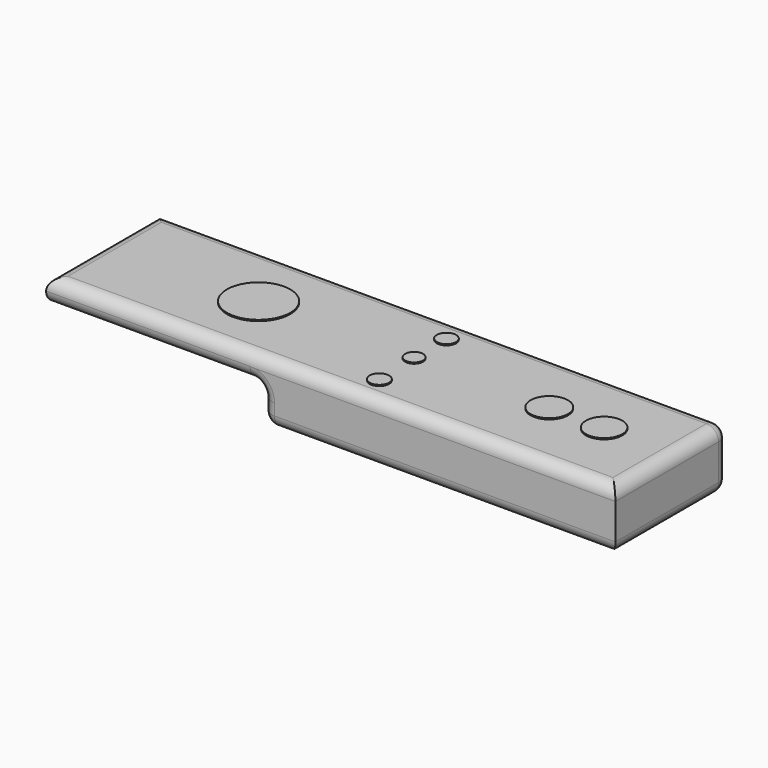
from build123d import *

# Parameters (mm, degrees)
F0_W          = 237.3272180557
F0_H          = 58.8164292276
F1_DEPTH      = 10
F2_W          = 147.2023129463
F2_H          = 58.8164292276
F3_DEPTH      = 15
F4_F1_R       = 5.08
F4_F2_R       = 5.08
F5_W          = 55.2143082023
F5_H          = 22.0865048468
F6_DEPTH      = 4
F7_T1_DEPTH   = 46.9058521388
F7_T3_DEPTH   = 80.0336554942
F9_R          = 13.2118644906
F10_DEPTH     = 0.5
F12_R         = 4.0488978151
F13_DEPTH     = 0.5
F12_R_2       = 3.7300649458
F12_R_3       = 4.0152102199
F12_R_4       = 7.8029945449
F12_R_5       = 7.5839402098
F14_T1_DEPTH  = 262.7272180557
F15_T1_DEPTH  = 66.4364292276
F15_T3_DEPTH  = 262.7272180557
F15_T5_DEPTH  = 14.84
F15_S9_W      = 5.08
F15_S9_H      = 5.08
F15_T10_DEPTH = 5.08
F15_T14_ANGLE = 89.9999999979
F16_T1_DEPTH  = 74.0564292276


# Not quite as in the source:
# - a fillet or chamfer that OpenCascade refuses, or shapes differently, is made with other operations: its cross-section is extruded or revolved along the edge and cut away or added


with BuildPart() as f1:
    # F0 (on Top) → F1 (new body)
    with BuildSketch(Plane.XY):
        Rectangle(F0_W, F0_H)
    extrude(amount=F1_DEPTH)

    # F2 (on face) → F3 (join)
    with BuildSketch(Plane(origin=(0, 0, 0), x_dir=(1, 0, 0), z_dir=(0, 0, -1))):
        with Locations((45.0624525547, 0)):
            Rectangle(F2_W, F2_H)
    extrude(amount=F3_DEPTH)

    # F4: fillet of radius 5.08 on 7 edges, made by hand

    # F4_f1
    f4_f1_edges = [f1.edges().sort_by_distance(p)[0] for p in [
        (-28.5387039185, 0, 0),
    ]]
    fillet(f4_f1_edges, radius=F4_F1_R)

    # F4_f2
    f4_f2_edges = [f1.edges().sort_by_distance(p)[0] for p in [
        (-28.5387039185, -29.4082146138, -10.04),
        (-28.5387039185, 29.4082146138, -10.04),
        (-28.5387039185, 0, -15),
        (45.0624525547, 29.4082146138, -15),
        (118.6636090279, 0, -15),
        (45.0624525547, -29.4082146138, -15),
        (-30.02660147, 29.4082146138, -1.4878975516),
        (-30.02660147, -29.4082146138, -1.4878975516),
    ]]
    fillet(f4_f2_edges, radius=F4_F2_R)

    # F5 (on face) → F6 (join)
    with BuildSketch(Plane(origin=(0, 0, 0), x_dir=(1, 0, 0), z_dir=(0, 0, -1))):
        with Locations((-83.400927484, 0)):
            Rectangle(F5_W, F5_H)
    extrude(amount=F6_DEPTH)

    # F7: fillet of radius 5.08 on 4 edges, made by hand

    # F7_s2 → F7_t1 (cut)
    with BuildSketch(Plane.XZ.offset(-23.4529260694)):
        with BuildLine():
            ThreePointArc((-55.7937733829, 0), (-57.5701673512, -2.8755530587), (-60.7576428413, -4))
            Line((-60.7576428413, -4), (-55.7937733829, -4))
            Line((-55.7937733829, -4), (-55.7937733829, 0))
        make_face()
        with BuildLine():
            ThreePointArc((-111.0080815852, 0), (-109.2316876169, -2.8755530587), (-106.0442121268, -4))
            Line((-106.0442121268, -4), (-111.0080815852, -4))
            Line((-111.0080815852, -4), (-111.0080815852, 0))
        make_face()
    extrude(amount=F7_T1_DEPTH, mode=Mode.SUBTRACT)

    # F7_s4 → F7_t3 (cut)
    with BuildSketch(Plane.YZ.offset(-123.4177552312)):
        with BuildLine():
            ThreePointArc((-11.0432524234, 0), (-9.2668584551, -2.8755530587), (-6.079382965, -4))
            Line((-6.079382965, -4), (-11.0432524234, -4))
            Line((-11.0432524234, -4), (-11.0432524234, 0))
        make_face()
        with BuildLine():
            ThreePointArc((11.0432524234, 0), (9.2668584551, -2.8755530587), (6.079382965, -4))
            Line((6.079382965, -4), (11.0432524234, -4))
            Line((11.0432524234, -4), (11.0432524234, 0))
        make_face()
    extrude(amount=F7_T3_DEPTH, mode=Mode.SUBTRACT)

    # F9 (on face) → F10 (join)
    with BuildSketch(Plane.XY.offset(10)):
        with Locations((-53.6077320576, 0)):
            Circle(F9_R)
    extrude(amount=F10_DEPTH)

    # F14: fillet of radius 5.08 on 1 edges, made by hand

    # F14_s2 → F14_t1 (cut)
    with BuildSketch(Plane.YZ.offset(-131.3636090279)):
        with BuildLine():
            ThreePointArc((24.3282146138, 10), (27.9203170622, 8.5121024484), (29.4082146138, 4.92))
            Line((29.4082146138, 4.92), (29.4082146138, 10))
            Line((29.4082146138, 10), (24.3282146138, 10))
        make_face()
    extrude(amount=F14_T1_DEPTH, mode=Mode.SUBTRACT)

    # F15: fillet of radius 5.08 on 2 edges, made by hand

    # F15_s2 → F15_t1 (cut)
    with BuildSketch(Plane.XZ.offset(-24.3282146138)):
        with BuildLine():
            ThreePointArc((118.6636090279, 4.92), (117.1757114763, 8.5121024484), (113.5836090279, 10))
            Line((113.5836090279, 10), (118.6636090279, 10))
            Line((118.6636090279, 10), (118.6636090279, 4.92))
        make_face()
    extrude(amount=F15_T1_DEPTH, mode=Mode.SUBTRACT)

    # F15_s4 → F15_t3 (cut)
    with BuildSketch(Plane.YZ.offset(-131.3636090279)):
        with BuildLine():
            ThreePointArc((-29.4082146138, 4.92), (-27.9203170622, 8.5121024484), (-24.3282146138, 10))
            Line((-24.3282146138, 10), (-29.4082146138, 10))
            Line((-29.4082146138, 10), (-29.4082146138, 4.92))
        make_face()
    extrude(amount=F15_T3_DEPTH, mode=Mode.SUBTRACT)

    # F15_s6 → F15_t5 (cut)
    with BuildSketch(Plane.XY.offset(-9.92)):
        with BuildLine():
            ThreePointArc((118.6636090279, 24.3282146138), (117.1757114763, 27.9203170622), (113.5836090279, 29.4082146138))
            Line((113.5836090279, 29.4082146138), (118.6636090279, 29.4082146138))
            Line((118.6636090279, 29.4082146138), (118.6636090279, 24.3282146138))
        make_face()
    extrude(amount=F15_T5_DEPTH, mode=Mode.SUBTRACT)


with BuildPart() as f13:
    # F12 (on face) → F13 (new body)
    with BuildSketch(Plane.XY.offset(10.5)):
        with Locations((12.0495855808, -19.1157609224)):
            Circle(F12_R)
    extrude(amount=F13_DEPTH)


with BuildPart() as f13b:
    # F12 (on face) → F13, piece 2 (new body)
    with BuildSketch(Plane.XY.offset(10.5)):
        with Locations((11.2095503137, 0)):
            Circle(F12_R_2)
    extrude(amount=F13_DEPTH)


with BuildPart() as f13c:
    # F12 (on face) → F13, piece 3 (new body)
    with BuildSketch(Plane.XY.offset(10.5)):
        with Locations((11.2095503137, 16.8793648481)):
            Circle(F12_R_3)
    extrude(amount=F13_DEPTH)


with BuildPart() as f13d:
    # F12 (on face) → F13, piece 4 (new body)
    with BuildSketch(Plane.XY.offset(10.5)):
        with Locations((67.5813481212, 0)):
            Circle(F12_R_4)
    extrude(amount=F13_DEPTH)


with BuildPart() as f13e:
    # F12 (on face) → F13, piece 5 (new body)
    with BuildSketch(Plane.XY.offset(10.5)):
        with Locations((90.4404297471, 0)):
            Circle(F12_R_5)
    extrude(amount=F13_DEPTH)


with BuildPart() as f15_tool8:
    # F15_s9 → F15_t10 (new body)
    with BuildSketch(Plane.YZ.offset(113.5836090279)):
        with Locations((26.8682146138, -12.46)):
            Rectangle(F15_S9_W, F15_S9_H)
    extrude(amount=F15_T10_DEPTH)

    # F15_s11 → F15_t12 (revolve, cut)
    with BuildSketch(Plane(origin=(113.5836090279, 24.3282146138, -9.92), x_dir=(0, -0.7071067812, 0.7071067812), z_dir=(0, 0.7071067812, 0.7071067812))):
        with BuildLine():
            ThreePointArc((0, -5.08), (5.08, 0), (0, 5.08))
            Line((0, 5.08), (0, -5.08))
        make_face()
    revolve(axis=Axis((113.5836090279, 24.3282146138, -9.92), (1, 0, 0)), mode=Mode.SUBTRACT)


with BuildPart() as f1_1:
    add(f1.part)

    # F15_t7: cut F15_tool8
    add(f15_tool8.part, mode=Mode.SUBTRACT)

    # F15_s13 → F15_t14 (revolve, cut)
    with BuildSketch(Plane.XZ.offset(-24.3282146137)):
        with BuildLine():
            ThreePointArc((118.6636090279, 4.92), (117.1757114763, 8.5121024484), (113.5836090279, 10))
            Line((113.5836090279, 10), (118.6636090279, 10))
            Line((118.6636090279, 10), (118.6636090279, 4.92))
        make_face()
    revolve(axis=Axis((118.6636090279, 24.3282146137, 4.9199999999), (-1, 0, 0)), revolution_arc=F15_T14_ANGLE, mode=Mode.SUBTRACT)

    # F16: fillet of radius 5.08 on 1 edges, made by hand

    # F16_s2 → F16_t1 (cut)
    with BuildSketch(Plane.XZ.offset(-37.0282146138)):
        with BuildLine():
            ThreePointArc((-118.6636090279, 4.92), (-117.1757114763, 8.5121024484), (-113.5836090279, 10))
            Line((-113.5836090279, 10), (-118.6636090279, 10))
            Line((-118.6636090279, 10), (-118.6636090279, 4.92))
        make_face()
    extrude(amount=F16_T1_DEPTH, mode=Mode.SUBTRACT)


solid = Compound([f13.part, f13b.part, f13c.part, f13d.part, f13e.part, f1_1.part])
